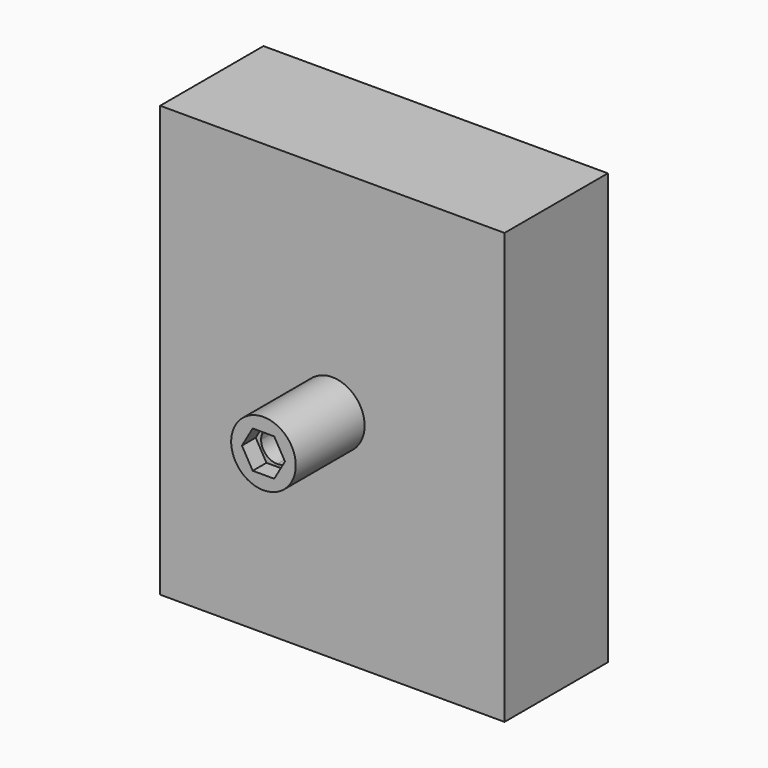
from build123d import *

# Parameters (mm, degrees)
F0_R         = 9.525
F1_DEPTH     = 25.4
F3_DEPTH     = 25.401
F4_DEPTH     = 11.0998
F6_DEPTH     = 5.08
F7_W         = 101.6
F7_H         = 127
F8_DEPTH     = 38.1
F9_T         = 2.54
F9_T3_DEPTH  = 10.16
F9_T5_DEPTH  = 11.43
F9_T7_DEPTH  = 11.43
F9_T9_DEPTH  = 11.43
F9_T11_DEPTH = 11.43
F9_T13_DEPTH = 11.43
F9_T15_DEPTH = 9.8425
F9_T17_DEPTH = 9.8425
F9_T19_DEPTH = 9.8425
F9_T21_DEPTH = 9.8425
F9_T23_DEPTH = 14.605
F9_T25_DEPTH = 16.1798
F9_T27_DEPTH = 14.605


# Not quite as in the source:
# - a shell that OpenCascade refuses in one call is made with other operations: the cavity is built on its own and cut out


with BuildPart() as f1:
    # F0 (on Front) → F1 (new body)
    with BuildSketch(Plane.XZ):
        Circle(F0_R)
    extrude(amount=F1_DEPTH)

    # F2 (on face) → F3 (cut, through all)
    with BuildSketch(Plane(origin=(0, 0, 0), x_dir=(-1, 0, 0), z_dir=(0, 1, 0))):
        with BuildLine():
            ThreePointArc((4.7625, 0), (3.3675960454, 3.3675960454), (0, 4.7625))
            ThreePointArc((0, 4.7625), (-3.3675960454, 3.3675960454), (-4.7625, 0))
            ThreePointArc((-4.7625, 0), (-3.3675960454, -3.3675960454), (0, -4.7625))
            ThreePointArc((0, -4.7625), (3.3675960454, -3.3675960454), (4.7625, 0))
        make_face()
    extrude(amount=-F3_DEPTH, mode=Mode.SUBTRACT)

    # F2 (on face) → F4 (cut)
    with BuildSketch(Plane(origin=(0, 0, 0), x_dir=(-1, 0, 0), z_dir=(0, 1, 0))):
        with BuildLine():
            Line((4.7625, 0), (4.7625, 4.7625))
            Line((4.7625, 4.7625), (0, 4.7625))
            ThreePointArc((0, 4.7625), (3.3675960454, 3.3675960454), (4.7625, 0))
        make_face()
        with BuildLine():
            ThreePointArc((-4.7625, 0), (-3.3675960454, 3.3675960454), (0, 4.7625))
            Line((0, 4.7625), (-4.7625, 4.7625))
            Line((-4.7625, 4.7625), (-4.7625, 0))
        make_face()
        with BuildLine():
            ThreePointArc((4.7625, 0), (3.3675960454, 3.3675960454), (0, 4.7625))
            ThreePointArc((0, 4.7625), (-3.3675960454, 3.3675960454), (-4.7625, 0))
            ThreePointArc((-4.7625, 0), (-3.3675960454, -3.3675960454), (0, -4.7625))
            ThreePointArc((0, -4.7625), (3.3675960454, -3.3675960454), (4.7625, 0))
        make_face()
        with BuildLine():
            Line((4.7625, -4.7625), (4.7625, 0))
            ThreePointArc((4.7625, 0), (3.3675960454, -3.3675960454), (0, -4.7625))
            Line((0, -4.7625), (4.7625, -4.7625))
        make_face()
        with BuildLine():
            ThreePointArc((0, -4.7625), (-3.3675960454, -3.3675960454), (-4.7625, 0))
            Line((-4.7625, 0), (-4.7625, -4.7625))
            Line((-4.7625, -4.7625), (0, -4.7625))
        make_face()
    extrude(amount=-F4_DEPTH, mode=Mode.SUBTRACT)

    # F5 (on face) → F6 (cut)
    with BuildSketch(Plane.XZ.offset(25.4)):
        Polygon((3.175, 5.499261314), (-3.175, 5.499261314), (-6.35, 0), (-3.175, -5.499261314), (3.175, -5.499261314), (6.35, 0), align=None)
    extrude(amount=-F6_DEPTH, mode=Mode.SUBTRACT)

    # F7 (on Front) → F8 (join)
    with BuildSketch(Plane.XZ):
        Rectangle(F7_W, F7_H)
    extrude(amount=-F8_DEPTH)

    # F9: shell of thickness 2.54, made by hand


with BuildPart() as f9_core1:
    # F9_t2: copy of F1
    add(f1.part)

    # the walls: a layer under each face that stays
    f9_faces = [f9_core1.faces().sort_by_distance(p)[0] for p in [
        (50.8, 19.05, 0),
        (0, 19.05, -63.5),
        (0, 19.05, 63.5),
        (-33.8666666667, 0, -42.3333333333),
        (-50.8, 19.05, 0),
        (-9.525, -12.7, 0),
        (-6.35, -25.4, -6.35),
        (0, -22.86, 5.499261314),
        (-4.7625, -22.86, 2.749630657),
        (-4.7625, -22.86, -2.749630657),
        (0, -22.86, -5.499261314),
        (4.7625, -22.86, -2.749630657),
        (4.7625, -22.86, 2.749630657),
        (-5.4428571429, -20.32, 0),
        (0, -15.7099, 4.7625),
        (-3.96875, -11.0998, -3.96875),
        (-3.96875, -11.0998, 3.96875),
        (3.96875, -11.0998, 3.96875),
        (3.96875, -11.0998, -3.96875),
        (-4.7625, -5.5499, 0),
        (0, -5.5499, -4.7625),
        (0, -5.5499, 4.7625),
        (4.7625, -5.5499, 0),
        (0, 0, 0),
    ]]
    thicken(f9_faces, amount=-F9_T, mode=Mode.SUBTRACT)

    # F9_s4 → F9_t3 (cut)
    with BuildSketch(Plane.XZ.offset(17.78)):
        Polygon((3.1530029547, 5.461161314), (3.175, 8.039261314), (4.6414696837, 8.039261314), (5.3747045256, 6.769261314), align=None)
        Polygon((-3.1530029547, 5.461161314), (-3.175, 8.039261314), (-4.6414696837, 8.039261314), (-5.3747045256, 6.769261314), align=None)
        Polygon((-6.3060059095, 0), (-8.5497045256, 1.27), (-9.2829393675, 0), (-8.5497045256, -1.27), align=None)
        Polygon((-3.1530029547, -5.461161314), (-5.3747045256, -6.769261314), (-4.6414696837, -8.039261314), (-3.175, -8.039261314), align=None)
        Polygon((3.1530029547, -5.461161314), (3.175, -8.039261314), (4.6414696837, -8.039261314), (5.3747045256, -6.769261314), align=None)
        Polygon((6.3060059095, 0), (8.5497045256, -1.27), (9.2829393675, 0), (8.5497045256, 1.27), align=None)
    extrude(amount=F9_T3_DEPTH, mode=Mode.SUBTRACT)

    # F9_s6 → F9_t5 (cut)
    with BuildSketch(Plane.YZ.offset(-5.715)):
        Polygon((-20.3454, 5.473861314), (-20.32, 8.039261314), (-17.78, 8.039261314), (-17.78, 5.499261314), align=None)
        Polygon((-20.3454, -5.473861314), (-20.32, -8.039261314), (-17.78, -8.039261314), (-17.78, -5.499261314), align=None)
    extrude(amount=F9_T5_DEPTH, mode=Mode.SUBTRACT)

    # F9_s8 → F9_t7 (cut)
    with BuildSketch(Plane(origin=(2.8575, 0, 4.9493351826), x_dir=(0, 1, 0), z_dir=(-0.5, 0, -0.8660254038))):
        Polygon((-20.3454, -5.473861314), (-20.32, -8.039261314), (-17.78, -8.039261314), (-17.78, -5.499261314), align=None)
    extrude(amount=F9_T7_DEPTH, mode=Mode.SUBTRACT)

    # F9_s10 → F9_t9 (cut)
    with BuildSketch(Plane(origin=(-2.8575, 0, 4.9493351826), x_dir=(0, 1, 0), z_dir=(0.5, 0, -0.8660254038))):
        Polygon((-20.3454, -5.473861314), (-20.32, -8.039261314), (-17.78, -8.039261314), (-17.78, -5.499261314), align=None)
    extrude(amount=F9_T9_DEPTH, mode=Mode.SUBTRACT)

    # F9_s12 → F9_t11 (cut)
    with BuildSketch(Plane(origin=(-2.8575, 0, -4.9493351826), x_dir=(0, 1, 0), z_dir=(0.5, 0, 0.8660254038))):
        Polygon((-20.3454, -5.473861314), (-20.32, -8.039261314), (-17.78, -8.039261314), (-17.78, -5.499261314), align=None)
    extrude(amount=F9_T11_DEPTH, mode=Mode.SUBTRACT)

    # F9_s14 → F9_t13 (cut)
    with BuildSketch(Plane(origin=(2.8575, 0, -4.9493351826), x_dir=(0, 1, 0), z_dir=(-0.5, 0, 0.8660254038))):
        Polygon((-20.3454, -5.473861314), (-20.32, -8.039261314), (-17.78, -8.039261314), (-17.78, -5.499261314), align=None)
    extrude(amount=F9_T13_DEPTH, mode=Mode.SUBTRACT)

    # F9_s16 → F9_t15 (cut)
    with BuildSketch(Plane.XY.offset(-7.3025)):
        Polygon((-4.7371, -11.0744), (-4.7625, -13.6398), (-7.3025, -13.6398), (-7.3025, -11.0998), align=None)
        Polygon((4.7371, -11.0744), (4.7625, -13.6398), (7.3025, -13.6398), (7.3025, -11.0998), align=None)
    extrude(amount=F9_T15_DEPTH, mode=Mode.SUBTRACT)

    # F9_s18 → F9_t17 (cut)
    with BuildSketch(Plane.YZ.offset(-7.3025)):
        Polygon((-11.0744, -4.7371), (-13.6398, -4.7625), (-13.6398, -7.3025), (-11.0998, -7.3025), align=None)
        Polygon((-11.0744, 4.7371), (-13.6398, 4.7625), (-13.6398, 7.3025), (-11.0998, 7.3025), align=None)
    extrude(amount=F9_T17_DEPTH, mode=Mode.SUBTRACT)

    # F9_s20 → F9_t19 (cut)
    with BuildSketch(Plane.XY.offset(-2.54)):
        Polygon((-4.7371, -11.0744), (-4.7625, -13.6398), (-7.3025, -13.6398), (-7.3025, -11.0998), align=None)
        Polygon((4.7371, -11.0744), (4.7625, -13.6398), (7.3025, -13.6398), (7.3025, -11.0998), align=None)
    extrude(amount=F9_T19_DEPTH, mode=Mode.SUBTRACT)

    # F9_s22 → F9_t21 (cut)
    with BuildSketch(Plane.YZ.offset(-2.54)):
        Polygon((-11.0744, 4.7371), (-13.6398, 4.7625), (-13.6398, 7.3025), (-11.0998, 7.3025), align=None)
        Polygon((-11.0744, -4.7371), (-13.6398, -4.7625), (-13.6398, -7.3025), (-11.0998, -7.3025), align=None)
    extrude(amount=F9_T21_DEPTH, mode=Mode.SUBTRACT)

    # F9_s24 → F9_t23 (cut)
    with BuildSketch(Plane.XY.offset(-7.3025)):
        Polygon((-4.7371, -0.0254), (-7.3025, 0), (-7.3025, 2.54), (-4.7625, 2.54), align=None)
        Polygon((4.7371, -0.0254), (7.3025, 0), (7.3025, 2.54), (4.7625, 2.54), align=None)
    extrude(amount=F9_T23_DEPTH, mode=Mode.SUBTRACT)

    # F9_s26 → F9_t25 (cut)
    with BuildSketch(Plane.XZ.offset(-2.54)):
        Polygon((-4.7371, -4.7371), (-7.3025, -4.7625), (-7.3025, -7.3025), (-4.7625, -7.3025), align=None)
        Polygon((-4.7371, 4.7371), (-7.3025, 4.7625), (-7.3025, 7.3025), (-4.7625, 7.3025), align=None)
        Polygon((4.7371, -4.7371), (4.7625, -7.3025), (7.3025, -7.3025), (7.3025, -4.7625), align=None)
        Polygon((4.7371, 4.7371), (4.7625, 7.3025), (7.3025, 7.3025), (7.3025, 4.7625), align=None)
    extrude(amount=F9_T25_DEPTH, mode=Mode.SUBTRACT)

    # F9_s28 → F9_t27 (cut)
    with BuildSketch(Plane.YZ.offset(-7.3025)):
        Polygon((-0.0254, -4.7371), (0, -7.3025), (2.54, -7.3025), (2.54, -4.7625), align=None)
        Polygon((-0.0254, 4.7371), (0, 7.3025), (2.54, 7.3025), (2.54, 4.7625), align=None)
    extrude(amount=F9_T27_DEPTH, mode=Mode.SUBTRACT)

    # F9_s29 → F9_t30 (revolve, cut)
    with BuildSketch(Plane.XY):
        Polygon((9.5504, -0.0254), (9.525, 2.54), (6.985, 2.54), (6.985, 0), align=None)
    revolve(axis=Axis((0, 0, 0), (0, -1, 0)), mode=Mode.SUBTRACT)


with BuildPart() as f1_1:
    add(f1.part)

    # what is left inside the walls is the cavity
    f9_cavity = [f9_core1.part.solids().sort_by_distance(p)[0] for p in [
        (0, 2.5654, -20.32),
    ]]
    add(f9_cavity, mode=Mode.SUBTRACT)


solid = f1_1.part
